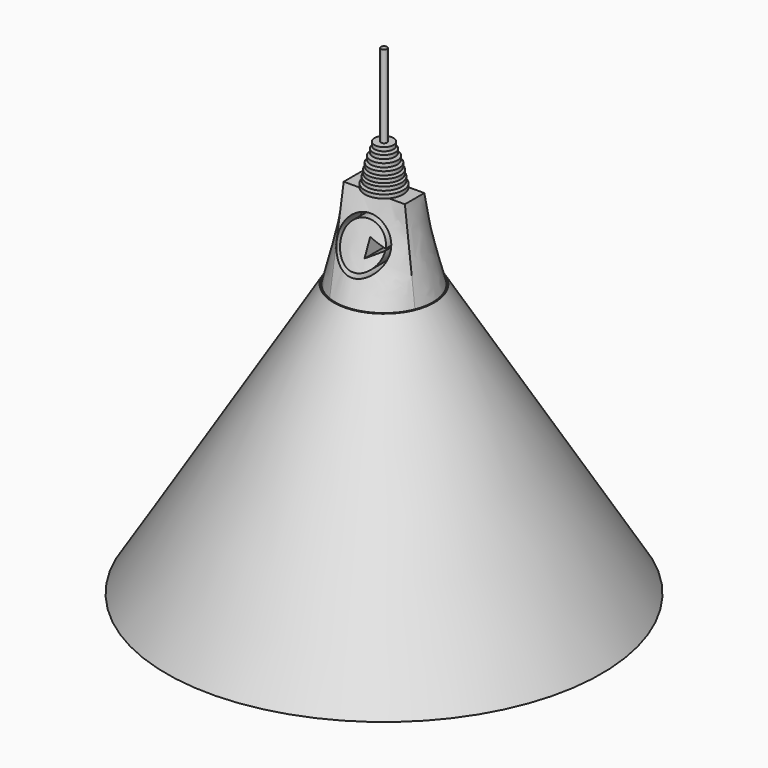
from build123d import *

# Parameters (mm, degrees)
F0_W     = 18.1671218015
F0_H     = 7.2170761414
F8_R     = 7.2452056649
F9_DEPTH = 12.7


# Not quite as in the source:
# - the arcs of a loft's sections are written as splines that run evenly, so that the points pair up as in the source's solid


with BuildPart() as f3:
    # F0 (on Top) → F3 section 0
    with BuildSketch(Plane.XY):
        Rectangle(F0_W, F0_H)
    # F2 (on offset) → F3 section 1
    with BuildSketch(Plane.XY.offset(-25.4)):
        with BuildLine():
            add(Edge.make_bspline(
                [(-13.4909534727, 5.359420138), (-14.1924999283, 3.593458458), (-14.5426369472, 1.6887002477), (-14.4873172157, -2.1113118661), (-14.0818822313, -4.0050706272), (-12.5765717848, -7.4946540977), (-11.4772885982, -9.0891058051), (-8.7511573067, -11.7370031821), (-7.125381818, -12.7894070172), (-5.359420138, -13.4909534727)],
                knots=[0, 0, 0, 0, 0.25, 0.25, 0.5, 0.5, 0.75, 0.75, 1, 1, 1, 1], degree=3))
            add(Edge.make_bspline(
                [(-5.359420138, -13.4909534727), (-3.593458458, -14.1924999283), (-1.6887002477, -14.5426369472), (2.1113118661, -14.4873172157), (4.0050706272, -14.0818822313), (7.4946540977, -12.5765717848), (9.0891058051, -11.4772885982), (11.7370031821, -8.7511573067), (12.7894070172, -7.125381818), (13.4909534727, -5.359420138)],
                knots=[0, 0, 0, 0, 0.25, 0.25, 0.5, 0.5, 0.75, 0.75, 1, 1, 1, 1], degree=3))
            add(Edge.make_bspline(
                [(13.4909534727, -5.359420138), (14.1924999283, -3.593458458), (14.5426369472, -1.6887002477), (14.4873172157, 2.1113118661), (14.0818822313, 4.0050706272), (12.5765717848, 7.4946540977), (11.4772885982, 9.0891058051), (8.7511573067, 11.7370031821), (7.125381818, 12.7894070172), (5.359420138, 13.4909534727)],
                knots=[0, 0, 0, 0, 0.25, 0.25, 0.5, 0.5, 0.75, 0.75, 1, 1, 1, 1], degree=3))
            add(Edge.make_bspline(
                [(5.359420138, 13.4909534727), (3.593458458, 14.1924999283), (1.6887002477, 14.5426369472), (-2.1113118661, 14.4873172157), (-4.0050706272, 14.0818822313), (-7.4946540977, 12.5765717848), (-9.0891058051, 11.4772885982), (-11.7370031821, 8.7511573067), (-12.7894070172, 7.125381818), (-13.4909534727, 5.359420138)],
                knots=[0, 0, 0, 0, 0.25, 0.25, 0.5, 0.5, 0.75, 0.75, 1, 1, 1, 1], degree=3))
        make_face()
    loft(ruled=True)

    # F6 (on Front) → F7 (revolve)
    with BuildSketch(Plane.XZ):
        Polygon((0.8841773961, 36.48737818), (0, 36.48737818), (0, -4.7170827165), (1.1227278737, -4.7170827165), (2.8959631454, -0.8159647114), (0.8841773961, -0.8159647114), (0.8841773961, 0), (5.6955757318, 0), (5.6955757318, 1.0931361467), (0.8841773961, 1.0931361467), (0.8841773961, 1.8148457166), (5.2144367946, 1.8148457166), (5.2144367946, 2.9079818632), (0.8841773961, 2.9079818632), (0.8841773961, 3.6296914332), (4.8776374315, 3.6296914332), (4.8776374315, 4.7228275798), (0.8841773961, 4.7228275798), (0.8841773961, 5.4445371497), (4.4927265262, 5.4445371497), (4.4927265262, 6.5376732964), (0.8841773961, 6.5376732964), (0.8841773961, 7.2593828663), (3.9634722052, 7.2593828663), (3.9634722052, 8.352519013), (0.8841773961, 8.352519013), (0.8841773961, 9.0742285829), (3.2898765639, 9.0742285829), (3.2898765639, 10.1673647296), (0.8841773961, 10.1673647296), (0.8841773961, 10.8890742995), (2.8368307394, 10.8890742995), (2.8368307394, 11.9822104461), (0.8841773961, 11.9822104461), align=None)
    revolve(axis=Axis((0, 0, 24.3908111006), (0, 0, -1)))

    # F8 (on Front) → F9 (cut)
    with BuildSketch(Plane.XZ):
        with Locations((0, -11.7249386385)):
            Circle(F8_R)
        with BuildLine():
            ThreePointArc((6.0419317468, -11.7540457542), (0, -17.7669404969), (-6.0419317468, -11.7540457542))
            ThreePointArc((-6.0419317468, -11.7540457542), (-6.0382916863, -11.5132313675), (-6.0250572559, -11.2727533669))
            ThreePointArc((-6.0250572559, -11.2727533669), (0, -5.6829367801), (6.0250572559, -11.2727533669))
            Line((6.0250572559, -11.2727533669), (1.7158846604, -9.4208233058))
            Line((1.7158846604, -9.4208233058), (1.7158846604, -14.2336934805))
            Line((1.7158846604, -14.2336934805), (6.0419317468, -11.7540457542))
        make_face(mode=Mode.SUBTRACT)
    extrude(amount=F9_DEPTH, mode=Mode.SUBTRACT)


with BuildPart() as f5:
    # F4 (on Front) → F5 (revolve)
    with BuildSketch(Plane.XZ):
        Polygon((-12.9464622587, -25.5154054612), (-14.9418804795, -25.2936929464), (-64.6056458354, -106.2190234661), (-62.1668025851, -106.2190234661), align=None)
    revolve(axis=Axis((0, 0, -68.527775351), (0, 0, 1)))


solid = Compound([f3.part, f5.part])
